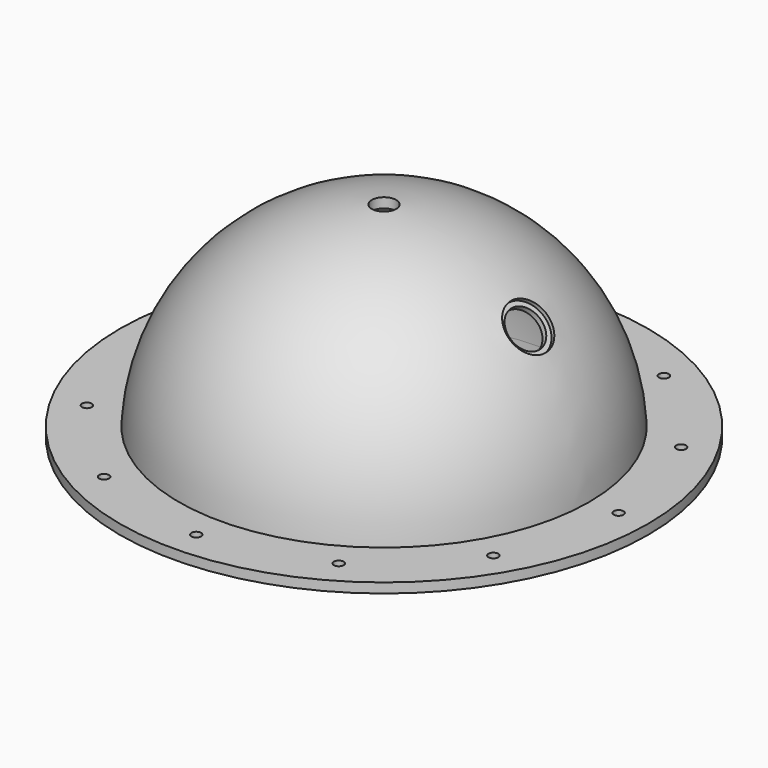
from build123d import *

# Parameters (mm, degrees)
F9_D            = 6.35
F9_COPIES_COUNT = 12


# Not quite as in the source:
# - a pattern or mirror of a feature is missing from the dataset's text; its kind, count and spacing are read off the source's solid


with BuildPart() as f1:
    # F0 (on Front) → F1 (revolve)
    with BuildSketch(Plane.XZ):
        with BuildLine():
            ThreePointArc((0, 127), (89.8025612107, 89.8025612107), (127, 0))
            Line((127, 0), (127, -6.35))
            Line((127, -6.35), (133.35, -6.35))
            Line((133.35, -6.35), (133.35, 0))
            Line((133.35, 0), (171.45, 0))
            Line((171.45, 0), (171.45, 6.35))
            Line((171.45, 6.35), (133.1987237176, 6.35))
            ThreePointArc((133.1987237176, 6.35), (92.0202423383, 96.5116443752), (0, 133.35))
            Line((0, 133.35), (0, 127))
        make_face()
    revolve(axis=Axis((0, 0, 13.3139304817), (0, 0, 1)))

    # F4 (on Front) → F5 (revolve, cut)
    with BuildSketch(Plane.XZ):
        with BuildLine():
            ThreePointArc((89.8025612107, 89.8025612107), (94.1857207861, 85.1941899427), (98.3326763457, 80.3721641036))
            Line((98.3326763457, 80.3721641036), (100.7753060106, 82.8147937685))
            Line((100.7753060106, 82.8147937685), (103.0203700409, 80.5697297382))
            Line((103.0203700409, 80.5697297382), (110.3632345412, 87.9125942385))
            Line((110.3632345412, 87.9125942385), (94.2926892712, 94.2926892712))
            Line((94.2926892712, 94.2926892712), (89.8025612107, 89.8025612107))
        make_face()
    f5 = revolve(axis=Axis((92.047625241, 0, 92.047625241), (0.7071067812, 0, 0.7071067812)), mode=Mode.SUBTRACT)

    # F5_copies: F5 across plane
    add(f5.mirror(Plane(origin=(0, 0, 0), x_dir=(0, 0, -1), z_dir=(-1, 0, 0))), mode=Mode.SUBTRACT)

    # F6 (on Front) → F7 (revolve, cut)
    with BuildSketch(Plane.XZ):
        with BuildLine():
            ThreePointArc((-7.9375, 126.7517104175), (-3.9706911856, 126.9379124277), (0, 127))
            Line((0, 127), (0, 133.35))
            ThreePointArc((0, 133.35), (-3.9705104321, 133.2908757076), (-7.9375, 133.1135552592))
            Line((-7.9375, 133.1135552592), (-7.9375, 126.7517104175))
        make_face()
    revolve(axis=Axis((0, 0, 130.175), (0, 0, 1)), mode=Mode.SUBTRACT)

    # F9 (through all)
    with Locations(Plane.XY.offset(6.35)):
        with Locations((0, -152.3243618588)):
            f9 = Hole(F9_D / 2)

    # F9_copies: F9 ×12 about axis
    f9_copies_axis = Axis((0, 0, 0), (0, 0, 1))
    for i in range(1, F9_COPIES_COUNT):
        add(f9.rotate(f9_copies_axis, i * 360 / F9_COPIES_COUNT), mode=Mode.SUBTRACT)


solid = f1.part
